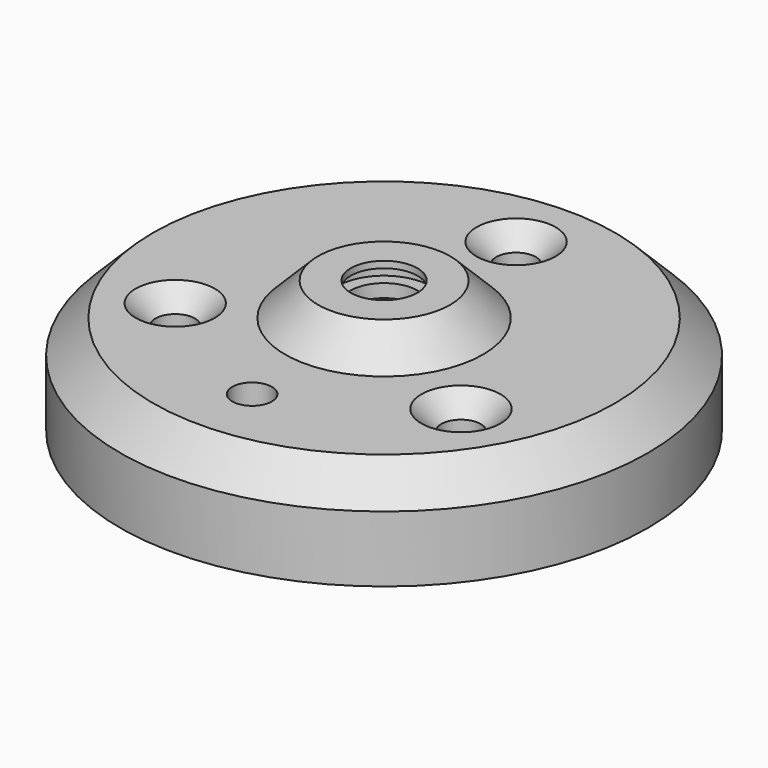
from build123d import *

# Parameters (mm, degrees)
F0_R           = 40
F1_DEPTH       = 15
F2_SIZE        = 5
F3_R           = 15
F4_DEPTH       = 5
F5_SIZE        = 4.99999
F7_D           = 6
F7_CSINK_D     = 12
F7_CSINK_ANGLE = 90
F8_D           = 10.1
F11_D          = 6


# Not quite as in the source:
# - a fillet or chamfer is up to 0.001 mm smaller than in the source, because OpenCascade refuses the exact size


with BuildPart() as f1:
    # F0 (on Top) → F1 (new body)
    with BuildSketch(Plane.XY):
        Circle(F0_R)
    extrude(amount=F1_DEPTH)

    # F2
    f2_edges = [f1.edges().sort_by_distance(p)[0] for p in [
        (-40, 0, 15),
    ]]
    chamfer(f2_edges, length=F2_SIZE)

    # F3 (on face) → F4 (join)
    with BuildSketch(Plane.XY.offset(15)):
        Circle(F3_R)
    extrude(amount=F4_DEPTH)

    # F5 (size 5 in the source; OpenCascade refuses exactly that, so slightly less here)
    f5_edges = [f1.edges().sort_by_distance(p)[0] for p in [
        (-15, 0, 20),
    ]]
    chamfer(f5_edges, length=F5_SIZE)

    # F7 (through all)
    with Locations(Plane.XY.offset(15)):
        with Locations((0, 25), (-21.6506350946, -12.5), (21.6506350946, -12.5)):
            CounterSinkHole(F7_D / 2, F7_CSINK_D / 2, counter_sink_angle=F7_CSINK_ANGLE)

    # F8 (through all)
    with Locations(Plane(origin=(0, 0, 0), x_dir=(1, 0, 0), z_dir=(0, 0, -1))):
        with Locations((0, 0)):
            Hole(F8_D / 2)

    # F9 (on Right) → F10 (revolve, cut)
    with BuildSketch(Plane.YZ):
        Polygon((7, 19), (0, 19), (0, 0), (7, 0), (7, 15), (5.1, 15), (5.1, 17), (7, 17), align=None)
    revolve(axis=Axis((0, 0, 9.5), (0, 0, 1)), mode=Mode.SUBTRACT)

    # F11 (through all)
    with Locations(Plane.XY.offset(15)):
        with Locations((0, -25)):
            Hole(F11_D / 2)


solid = f1.part
